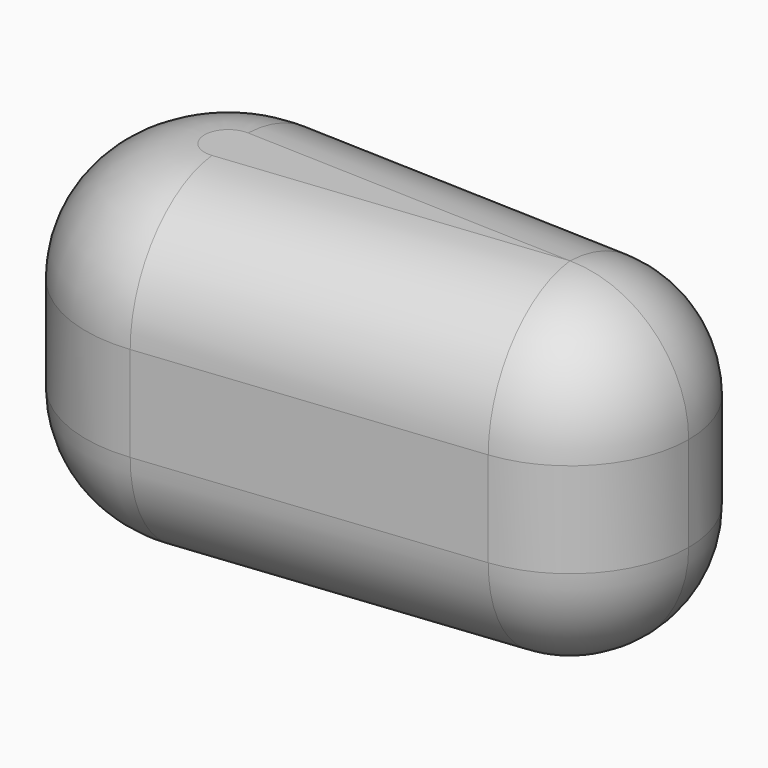
from build123d import *

# Parameters (mm, degrees)
F1_R     = 0.05
F2_DEPTH = 5.6
F3_DEPTH = 0.05
F4_R     = 4


# Not quite as in the source:
# - a feature names something its author has since deleted; it is built from what else it names


with BuildPart() as f2:
    # F1 (on Top) → F2 (new body, symmetric)
    with BuildSketch(Plane.XY):
        with BuildLine():
            ThreePointArc((-14.6792257551, -9.5724401661), (-11.6217612132, -8.0073805729), (-10.3928548637, -4.8))
            ThreePointArc((-10.3928548637, -4.8), (-11.7385887293, -1.4671265442), (-15.0212071439, -0.003070038))
            ThreePointArc((-15.0212071439, -0.003070038), (-19.9897926624, -4.9714285714), (-14.6792257551, -9.5724401661))
        make_face()
        with Locations((-15.1928548637, -4.8)):
            Circle(F1_R, mode=Mode.SUBTRACT)
        with BuildLine():
            ThreePointArc((-15.0212071439, -0.003070038), (-11.7385887293, -1.4671265442), (-10.3928548637, -4.8))
            ThreePointArc((-10.3928548637, -4.8), (-11.6217612132, -8.0073805729), (-14.6792257551, -9.5724401661))
            Line((-14.6792257551, -9.5724401661), (-3.5719757428, -8.3770334717))
            ThreePointArc((-3.5719757428, -8.3770334717), (-7.9974481656, -4.5428571429), (-3.8569602335, -0.402558365))
            Line((-3.8569602335, -0.402558365), (-15.0212071439, -0.003070038))
        make_face()
        with BuildLine():
            ThreePointArc((0, -4.4), (-1.121444888, -1.6226054535), (-3.8569602335, -0.402558365))
            ThreePointArc((-3.8569602335, -0.402558365), (-7.9974481656, -4.5428571429), (-3.5719757428, -8.3770334717))
            ThreePointArc((-3.5719757428, -8.3770334717), (-1.0240886246, -7.0728171441), (0, -4.4))
        make_face()
        with Locations((-4, -4.4)):
            Circle(F1_R, mode=Mode.SUBTRACT)
        with Locations((-15.1928548637, -4.8)):
            Circle(F1_R)
        with Locations((-4, -4.4)):
            Circle(F1_R)
    extrude(amount=F2_DEPTH, both=True)

    # F1 (on Top) → F3 (cut, symmetric)
    with BuildSketch(Plane.XY):
        with Locations((-15.1928548637, -4.8)):
            Circle(F1_R)
        with Locations((-4, -4.4)):
            Circle(F1_R)
    extrude(amount=F3_DEPTH, both=True, mode=Mode.SUBTRACT)

    # F4
    f4_edges = [f2.edges().sort_by_distance(p)[0] for p in [
        (-19.989793, -4.971429, 5.6),
        (-9.125601, -8.974737, 5.6),
        (-0.002552, -4.257143, 5.6),
        (-9.439084, -0.202814, 5.6),
        (-19.989793, -4.971429, -5.6),
        (-9.125601, -8.974737, -5.6),
        (-0.002552, -4.257143, -5.6),
        (-9.439084, -0.202814, -5.6),
    ]]
    fillet(f4_edges, radius=F4_R)


solid = f2.part
